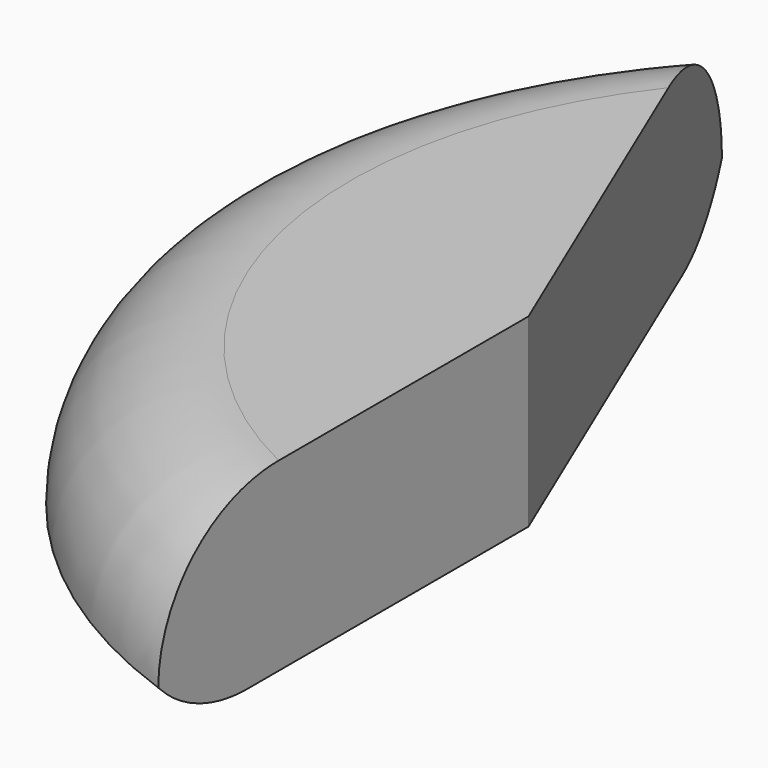
from build123d import *

# Parameters (mm, degrees)
F1_DEPTH    = 2.54
F2_R        = 1.905
F3_T2_ANGLE = 165.8998366825


# Not quite as in the source:
# - a fillet or chamfer that OpenCascade refuses, or shapes differently, is made with other operations: its cross-section is extruded or revolved along the edge and cut away or added


with BuildPart() as f1:
    # F0 (on Top) → F1 (new body)
    with BuildSketch(Plane.XY):
        with BuildLine():
            Line((0, -6.35), (0, 0))
            Line((0, 0), (-2.9618976002, 7.0207950124))
            ThreePointArc((-2.9618976002, 7.0207950124), (-5.171443726, -0.4821206784), (0, -6.35))
        make_face()
    extrude(amount=F1_DEPTH)

    # F2
    f2_edges = [f1.edges().sort_by_distance(p)[0] for p in [
        (-5.171444, -0.482121, 2.54),
    ]]
    fillet(f2_edges, radius=F2_R)

    # F3: fillet of radius 1.905 on 1 edges, made by hand

    # F3_s1 → F3_t2 (revolve, cut)
    with BuildSketch(Plane(origin=(2.823536152, 1.0021154347, 0), x_dir=(0, 0, 1), z_dir=(0.942405074, 0.3344737307, 0))):
        with BuildLine():
            ThreePointArc((0.635, -8.3742865468), (0.1659808799, -7.7320963745), (0, -6.9543833811))
            Line((0, -6.9543833811), (0, -8.3742865468))
            Line((0, -8.3742865468), (0.635, -8.3742865468))
        make_face()
    revolve(axis=Axis((2.7291622611, 1.2680210216, 0), (0, 0, 1)), revolution_arc=F3_T2_ANGLE, mode=Mode.SUBTRACT)


solid = f1.part
